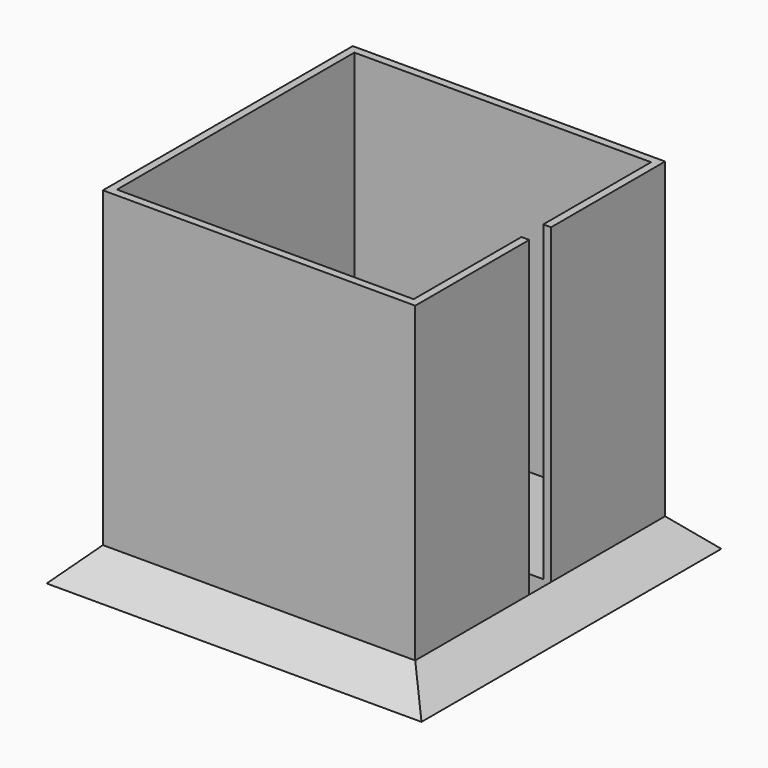
from build123d import *

# Parameters (mm, degrees)
F0_W     = 5.08
F0_H     = 4.445
F1_DEPTH = 5.08
F2_DEPTH = 55.88
F4_SIZE  = 5.07999


# Not quite as in the source:
# - a fillet or chamfer is up to 0.001 mm smaller than in the source, because OpenCascade refuses the exact size


with BuildPart() as f1:
    # F0 (on Top) → F1 (new body)
    with BuildSketch(Plane.XY):
        Polygon((0, -50.8), (0, 0), (50.8, 0), (50.8, -23.1775), (55.88, -23.1775), (55.88, 5.08), (-5.08, 5.08), (-5.08, -55.88), (55.88, -55.88), (55.88, -27.6225), (50.8, -27.6225), (50.8, -50.8), align=None)
        with Locations((53.34, -25.4)):
            Rectangle(F0_W, F0_H)
        Polygon((28.8019571453, -23.1775), (49.53, -23.1775), (49.53, -1.27), (1.27, -1.27), (1.27, -49.53), (49.53, -49.53), (49.53, -27.6225), (28.8019571453, -27.6225), (28.8019571453, -30.439995), (21.8463055789, -30.439995), (21.8463055789, -20.360005), (28.8019571453, -20.360005), align=None)
        Polygon((50.8, 0), (0, 0), (0, -50.8), (50.8, -50.8), (50.8, -27.6225), (49.53, -27.6225), (49.53, -49.53), (1.27, -49.53), (1.27, -1.27), (49.53, -1.27), (49.53, -23.1775), (50.8, -23.1775), align=None)
    extrude(amount=F1_DEPTH)

    # F0 (on Top) → F2 (join)
    with BuildSketch(Plane.XY):
        Polygon((50.8, 0), (0, 0), (0, -50.8), (50.8, -50.8), (50.8, -27.6225), (49.53, -27.6225), (49.53, -49.53), (1.27, -49.53), (1.27, -1.27), (49.53, -1.27), (49.53, -23.1775), (50.8, -23.1775), align=None)
    extrude(amount=F2_DEPTH)

    # F4 (size 5.08 in the source; OpenCascade refuses exactly that, so slightly less here)
    f4_edges = [f1.edges().sort_by_distance(p)[0] for p in [
        (-5.08, -25.4, 5.08),
        (25.4, -55.88, 5.08),
        (55.88, -25.4, 5.08),
        (25.4, 5.08, 5.08),
    ]]
    chamfer(f4_edges, length=F4_SIZE)


solid = f1.part
